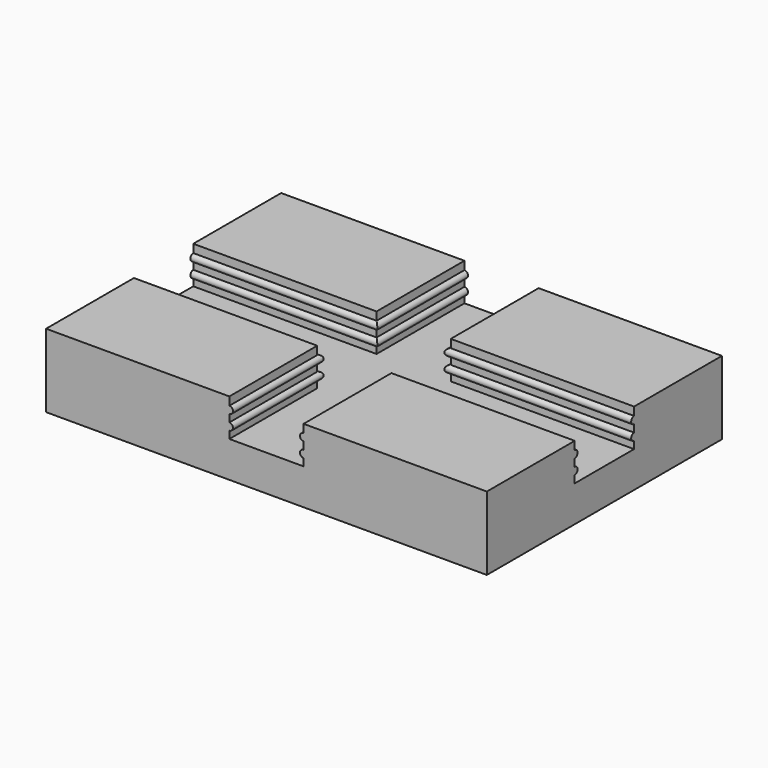
from build123d import *

# Parameters (mm, degrees)
F0_W     = 76.2
F0_H     = 50.8
F1_DEPTH = 12.7
F3_DEPTH = 50.801
F5_DEPTH = 76.201
F6_R     = 1.27
F7_DEPTH = 12.701


# Not quite as in the source:
# - a feature names something its author has since deleted; it is built from what else it names


with BuildPart() as f1:
    # F0 (on Top) → F1 (new body)
    with BuildSketch(Plane.XY):
        Rectangle(F0_W, F0_H)
    extrude(amount=F1_DEPTH)

    # F2 (on face) → F3 (cut, through all)
    with BuildSketch(Plane.XZ.offset(25.4)):
        with BuildLine():
            Line((6.4135, 12.7), (-6.4135, 12.7))
            Line((-6.4135, 12.7), (-6.4135, 11.2776))
            ThreePointArc((-6.4135, 11.2776), (-5.7912, 10.6553), (-6.4135, 10.033))
            Line((-6.4135, 10.033), (-6.4135, 8.7376))
            ThreePointArc((-6.4135, 8.7376), (-5.7912, 8.1153), (-6.4135, 7.493))
            Line((-6.4135, 7.493), (-6.4135, 6.223))
            Line((-6.4135, 6.223), (6.4135, 6.223))
            Line((6.4135, 6.223), (6.4135, 7.493))
            ThreePointArc((6.4135, 7.493), (5.7912, 8.1153), (6.4135, 8.7376))
            Line((6.4135, 8.7376), (6.4135, 10.033))
            ThreePointArc((6.4135, 10.033), (5.7912, 10.6553), (6.4135, 11.2776))
            Line((6.4135, 11.2776), (6.4135, 12.7))
        make_face()
    extrude(amount=-F3_DEPTH, mode=Mode.SUBTRACT)

    # F4 (on face) → F5 (cut, through all)
    with BuildSketch(Plane.YZ.offset(38.1)):
        with BuildLine():
            Line((6.4135, 12.7), (-6.4135, 12.7))
            Line((-6.4135, 12.7), (-6.4135, 11.2776))
            ThreePointArc((-6.4135, 11.2776), (-5.7912, 10.6553), (-6.4135, 10.033))
            Line((-6.4135, 10.033), (-6.4135, 8.7376))
            ThreePointArc((-6.4135, 8.7376), (-5.7912, 8.1153), (-6.4135, 7.493))
            Line((-6.4135, 7.493), (-6.4135, 6.223))
            Line((-6.4135, 6.223), (6.4135, 6.223))
            Line((6.4135, 6.223), (6.4135, 7.493))
            ThreePointArc((6.4135, 7.493), (5.7912, 8.1153), (6.4135, 8.7376))
            Line((6.4135, 8.7376), (6.4135, 10.033))
            ThreePointArc((6.4135, 10.033), (5.7912, 10.6553), (6.4135, 11.2776))
            Line((6.4135, 11.2776), (6.4135, 12.7))
        make_face()
    extrude(amount=-F5_DEPTH, mode=Mode.SUBTRACT)

    # F6 (on Top) → F7 (cut, through all)
    with BuildSketch(Plane.XY):
        Circle(F6_R)
    extrude(amount=F7_DEPTH, mode=Mode.SUBTRACT)


solid = f1.part
